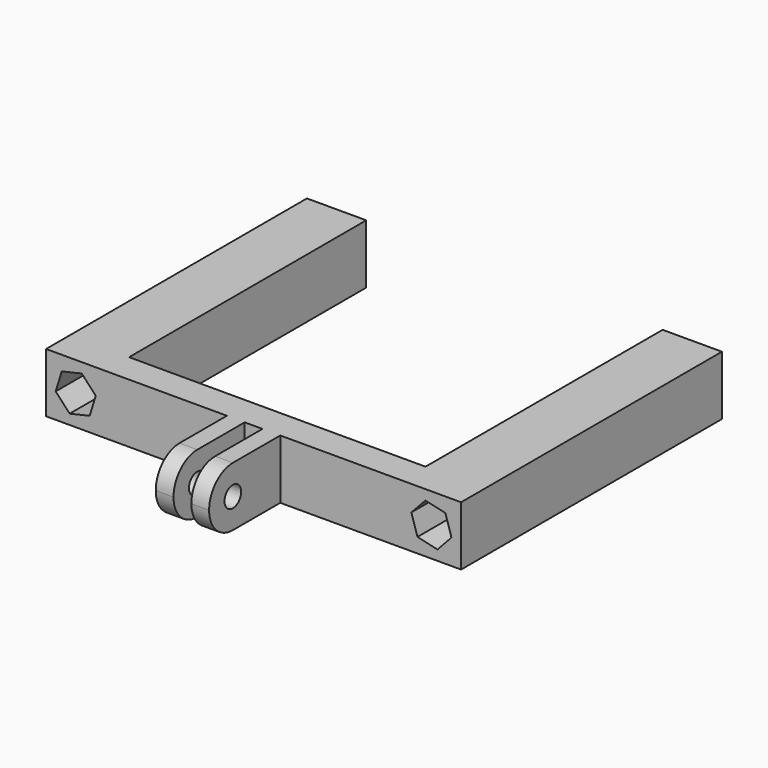
from build123d import *

# Parameters (mm, degrees)
F0_W      = 10
F0_H      = 10
F0_R      = 2.18110555
F1_DEPTH  = 50
F2_R      = 2.18110555
F2_R_2    = 1.75
F3_DEPTH  = 45
F4_W      = 35
F4_H      = 10
F5_DEPTH  = 5
F7_W      = 3
F7_H      = 10
F8_DEPTH  = 15
F9_R      = 1.75
F10_DEPTH = 39.501


# Not quite as in the source:
# - a feature names something its author has since deleted; it is built from what else it names


with BuildPart() as f1:
    # F0 (on Front) → F1 (new body)
    with BuildSketch(Plane.XZ):
        with Locations((-24.531819516, -5.3058740483)):
            Rectangle(F0_W, F0_H)
        with Locations((-24.531819516, -5.3058740483)):
            Circle(F0_R, mode=Mode.SUBTRACT)
    extrude(amount=-F1_DEPTH)

    # F2 (on face) → F3 (cut)
    with BuildSketch(Plane.XZ):
        Polygon((-22.1752951329, -7.844927579), (-21.1546724653, -4.5345908332), (-23.5111968485, -1.9955373025), (-26.8883438992, -2.7668205176), (-27.9089665667, -6.0771572634), (-25.5524421836, -8.6162107941), align=None)
        with Locations((-24.531819516, -5.3058740483)):
            Circle(F2_R, mode=Mode.SUBTRACT)
        Polygon((36.9860127402, -8.419743866), (38.9237869783, -5.5483276646), (37.4059547221, -2.4344578468), (33.9503482277, -2.1920042306), (32.0125739896, -5.063420432), (33.5304062458, -8.1772902498), align=None)
        with Locations((35.468180484, -5.3058740483)):
            Circle(F2_R_2, mode=Mode.SUBTRACT)
    extrude(amount=-F3_DEPTH, mode=Mode.SUBTRACT)

    # F4 (on face) → F5 (join)
    with BuildSketch(Plane.XZ):
        with Locations((-12.031819516, -5.3058740483)):
            Rectangle(F4_W, F4_H)
        Polygon((-22.1752951329, -7.844927579), (-25.5524421836, -8.6162107941), (-27.9089665667, -6.0771572634), (-26.8883438992, -2.7668205176), (-23.5111968485, -1.9955373025), (-21.1546724653, -4.5345908332), align=None, mode=Mode.SUBTRACT)
    extrude(amount=F5_DEPTH)

    # F6: F1 across face


with BuildPart() as f1_1:
    add(f1.part)
    add(f1.part.mirror(Plane(origin=(5.468180484, -2.5, -5.3058740483), x_dir=(0, 1, 0), z_dir=(1, 0, 0))))

    # F7 (on face) → F8 (join)
    with BuildSketch(Plane.XZ.offset(5)):
        with Locations((8.468180484, -5.3058740483)):
            Rectangle(F7_W, F7_H)
        with Locations((2.468180484, -5.3058740483)):
            Rectangle(F7_W, F7_H)
    extrude(amount=F8_DEPTH)

    # F9 (on face) → F10 (cut, through all)
    with BuildSketch(Plane.YZ.offset(9.968180484)):
        with BuildLine():
            ThreePointArc((-20, -5.3058740483), (-18.5355339059, -1.7703401424), (-15, -0.3058740483))
            Line((-15, -0.3058740483), (-20, -0.3058740483))
            Line((-20, -0.3058740483), (-20, -5.3058740483))
        make_face()
        with Locations((-15, -5.3058740483)):
            Circle(F9_R)
        with BuildLine():
            ThreePointArc((-15, -10.3058740483), (-18.5355339059, -8.8414079542), (-20, -5.3058740483))
            Line((-20, -5.3058740483), (-20, -10.3058740483))
            Line((-20, -10.3058740483), (-15, -10.3058740483))
        make_face()
    extrude(amount=-F10_DEPTH, mode=Mode.SUBTRACT)


solid = f1_1.part
